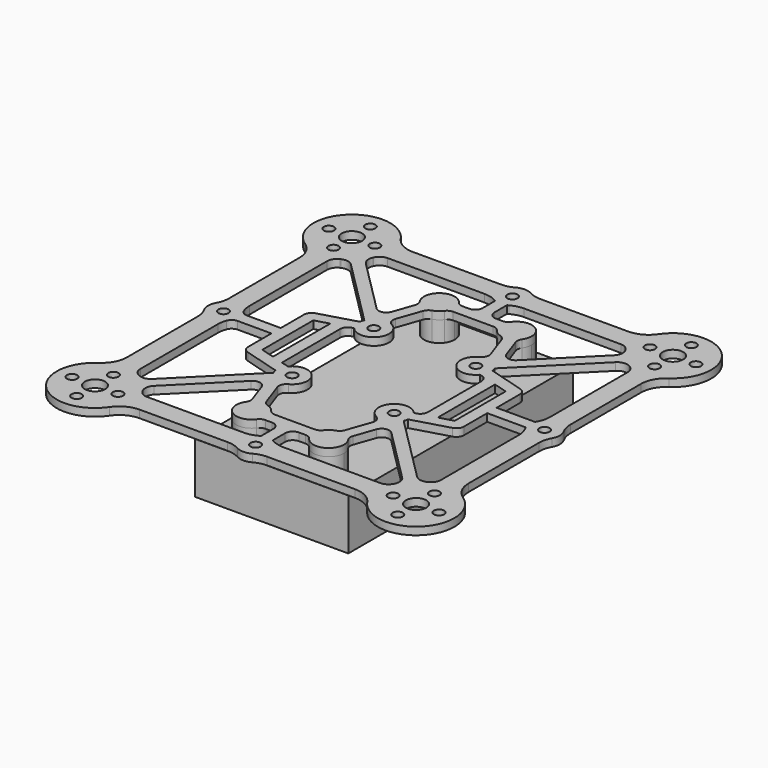
from build123d import *

# Parameters (mm, degrees)
F1_R     = 1
F1_R_2   = 2
F2_DEPTH = 1.5
F4_DEPTH = 4
F5_W     = 30
F5_H     = 55
F5_R     = 3
F6_DEPTH = 10


with BuildPart() as f2:
    # F1 (on Top) → F2 (new body)
    with BuildSketch(Plane.XY):
        with BuildLine():
            ThreePointArc((-33.4662517628, -21.1100941742), (-34.0503713296, -23.4553020541), (-35.6662517628, -25.2525572096))
            ThreePointArc((-35.6662517628, -25.2525572096), (-36.7695526217, -36.7695526217), (-25.2525572096, -35.6662517628))
            ThreePointArc((-25.2525572096, -35.6662517628), (-23.4553020541, -34.0503713296), (-21.1100941742, -33.4662517628))
            Line((-21.1100941742, -33.4662517628), (-3.8729833462, -33.4662517628))
            ThreePointArc((-3.8729833462, -33.4662517628), (-2.6229833462, -33.62502258), (-1.4523687548, -34.0912517628))
            ThreePointArc((-1.4523687548, -34.0912517628), (0, -34.4662517628), (1.4523687548, -34.0912517628))
            ThreePointArc((1.4523687548, -34.0912517628), (2.6229833462, -33.62502258), (3.8729833462, -33.4662517628))
            Line((3.8729833462, -33.4662517628), (21.1100941742, -33.4662517628))
            ThreePointArc((21.1100941742, -33.4662517628), (23.4553020541, -34.0503713296), (25.2525572096, -35.6662517628))
            ThreePointArc((25.2525572096, -35.6662517628), (36.7695526217, -36.7695526217), (35.6662517628, -25.2525572096))
            ThreePointArc((35.6662517628, -25.2525572096), (34.0503713296, -23.4553020541), (33.4662517628, -21.1100941742))
            Line((33.4662517628, -21.1100941742), (33.4662517628, -3.8729833462))
            ThreePointArc((33.4662517628, -3.8729833462), (33.62502258, -2.6229833462), (34.0912517628, -1.4523687548))
            ThreePointArc((34.0912517628, -1.4523687548), (34.4662517628, 0), (34.0912517628, 1.4523687548))
            ThreePointArc((34.0912517628, 1.4523687548), (33.62502258, 2.6229833462), (33.4662517628, 3.8729833462))
            Line((33.4662517628, 3.8729833462), (33.4662517628, 21.1100941742))
            ThreePointArc((33.4662517628, 21.1100941742), (34.0503713296, 23.4553020541), (35.6662517628, 25.2525572096))
            ThreePointArc((35.6662517628, 25.2525572096), (36.7695526217, 36.7695526217), (25.2525572096, 35.6662517628))
            ThreePointArc((25.2525572096, 35.6662517628), (23.4553020541, 34.0503713296), (21.1100941742, 33.4662517628))
            Line((21.1100941742, 33.4662517628), (3.8729833462, 33.4662517628))
            ThreePointArc((3.8729833462, 33.4662517628), (2.6229833462, 33.62502258), (1.4523687548, 34.0912517628))
            ThreePointArc((1.4523687548, 34.0912517628), (0, 34.4662517628), (-1.4523687548, 34.0912517628))
            ThreePointArc((-1.4523687548, 34.0912517628), (-2.6229833462, 33.62502258), (-3.8729833462, 33.4662517628))
            Line((-3.8729833462, 33.4662517628), (-21.1100941742, 33.4662517628))
            ThreePointArc((-21.1100941742, 33.4662517628), (-23.4553020541, 34.0503713296), (-25.2525572096, 35.6662517628))
            ThreePointArc((-25.2525572096, 35.6662517628), (-36.7695526217, 36.7695526217), (-35.6662517628, 25.2525572096))
            ThreePointArc((-35.6662517628, 25.2525572096), (-34.0503713296, 23.4553020541), (-33.4662517628, 21.1100941742))
            Line((-33.4662517628, 21.1100941742), (-33.4662517628, 3.8729833462))
            ThreePointArc((-33.4662517628, 3.8729833462), (-33.62502258, 2.6229833462), (-34.0912517628, 1.4523687548))
            ThreePointArc((-34.0912517628, 1.4523687548), (-34.4662517628, 0), (-34.0912517628, -1.4523687548))
            ThreePointArc((-34.0912517628, -1.4523687548), (-33.62502258, -2.6229833462), (-33.4662517628, -3.8729833462))
            Line((-33.4662517628, -3.8729833462), (-33.4662517628, -21.1100941742))
        make_face()
        with Locations((-31.4662517628, -35.9662517628)):
            Circle(F1_R, mode=Mode.SUBTRACT)
        with Locations((-35.9662517628, -31.4662517628)):
            Circle(F1_R, mode=Mode.SUBTRACT)
        with Locations((-31.4662517628, -31.4662517628)):
            Circle(F1_R_2, mode=Mode.SUBTRACT)
        with Locations((-26.9662517628, -31.4662517628)):
            Circle(F1_R, mode=Mode.SUBTRACT)
        with Locations((-31.4662517628, -26.9662517628)):
            Circle(F1_R, mode=Mode.SUBTRACT)
        with BuildLine():
            ThreePointArc((-22.849407793, -29.4662517628), (-23.9254629667, -29.1521062236), (-24.6634802077, -28.308357026))
            ThreePointArc((-24.6634802077, -28.308357026), (-24.6838554075, -28.2648302537), (-24.7045091049, -28.2214349377))
            ThreePointArc((-24.7045091049, -28.2214349377), (-24.8728885591, -27.0197800467), (-24.3155912919, -25.9419368886))
            Line((-24.3155912919, -25.9419368886), (-13.7338277743, -15.360173371))
            ThreePointArc((-13.7338277743, -15.360173371), (-12.3402923362, -14.9582351505), (-11.257957598, -15.9236608934))
            Line((-11.257957598, -15.9236608934), (-9.8435524525, -19.9497880645))
            ThreePointArc((-9.8435524525, -19.9497880645), (-9.7719536477, -20.6454539498), (-10.0235391122, -21.2979738092))
            ThreePointArc((-10.0235391122, -21.2979738092), (-9.2875900594, -25.4477577388), (-5.1284504101, -24.7666666667))
            ThreePointArc((-5.1284504101, -24.7666666667), (-4.5962029293, -24.3130258043), (-3.9161294039, -24.15))
            Line((-3.9161294039, -24.15), (-2.65, -24.15))
            ThreePointArc((-2.65, -24.15), (-1.5893398282, -24.5893398282), (-1.15, -25.65))
            Line((-1.15, -25.65), (-1.15, -28.6954215623))
            ThreePointArc((-1.15, -28.6954215623), (-1.3032257655, -28.7641039867), (-1.4523687548, -28.8412517628))
            ThreePointArc((-1.4523687548, -28.8412517628), (-2.6229833462, -29.3074809456), (-3.8729833462, -29.4662517628))
            Line((-3.8729833462, -29.4662517628), (-22.849407793, -29.4662517628))
        make_face(mode=Mode.SUBTRACT)
        with BuildLine():
            ThreePointArc((-28.308357026, -24.6634802077), (-29.1521062236, -23.9254629667), (-29.4662517628, -22.849407793))
            Line((-29.4662517628, -22.849407793), (-29.4662517628, -3.8729833462))
            ThreePointArc((-29.4662517628, -3.8729833462), (-29.3868269069, -2.9853233599), (-29.1510756623, -2.1258642802))
            ThreePointArc((-29.1510756623, -2.1258642802), (-28.6011389892, -1.4178872658), (-27.7456284924, -1.15))
            Line((-27.7456284924, -1.15), (-21.15, -1.15))
            Line((-21.15, -1.15), (-21.15, -6.8384922452))
            ThreePointArc((-21.15, -6.8384922452), (-20.8492479119, -7.7394941575), (-20.0675940722, -8.2791917944))
            Line((-20.0675940722, -8.2791917944), (-12.9814446691, -10.3331481431))
            ThreePointArc((-12.9814446691, -10.3331481431), (-12.9055182091, -10.7469698366), (-12.7724456227, -11.1461000259))
            Line((-12.7724456227, -11.1461000259), (-25.9419368886, -24.3155912919))
            ThreePointArc((-25.9419368886, -24.3155912919), (-27.0197800467, -24.8728885591), (-28.2214349377, -24.7045091049))
            ThreePointArc((-28.2214349377, -24.7045091049), (-28.2648302537, -24.6838554075), (-28.308357026, -24.6634802077))
        make_face(mode=Mode.SUBTRACT)
        with Locations((-10, -10)):
            Circle(F1_R, mode=Mode.SUBTRACT)
        Polygon((-18.85, 6.237447605), (-16.15, 7.0200563006), (-16.15, -7.0200563006), (-18.85, -6.237447605), align=None, mode=Mode.SUBTRACT)
        with Locations((0, -31.4662517628)):
            Circle(F1_R, mode=Mode.SUBTRACT)
        with BuildLine():
            ThreePointArc((24.6634802077, -28.308357026), (23.9254629667, -29.1521062236), (22.849407793, -29.4662517628))
            Line((22.849407793, -29.4662517628), (3.8729833462, -29.4662517628))
            ThreePointArc((3.8729833462, -29.4662517628), (2.6229833462, -29.3074809456), (1.4523687548, -28.8412517628))
            ThreePointArc((1.4523687548, -28.8412517628), (1.3032257655, -28.7641039867), (1.15, -28.6954215623))
            Line((1.15, -28.6954215623), (1.15, -25.65))
            ThreePointArc((1.15, -25.65), (1.5893398282, -24.5893398282), (2.65, -24.15))
            Line((2.65, -24.15), (3.9161294039, -24.15))
            ThreePointArc((3.9161294039, -24.15), (4.5962029293, -24.3130258043), (5.1284504101, -24.7666666667))
            ThreePointArc((5.1284504101, -24.7666666667), (9.2875900594, -25.4477577388), (10.0235391122, -21.2979738092))
            ThreePointArc((10.0235391122, -21.2979738092), (9.7719536477, -20.6454539498), (9.8435524525, -19.9497880645))
            Line((9.8435524525, -19.9497880645), (11.257957598, -15.9236608934))
            ThreePointArc((11.257957598, -15.9236608934), (12.3402923362, -14.9582351505), (13.7338277743, -15.360173371))
            Line((13.7338277743, -15.360173371), (24.3155912919, -25.9419368886))
            ThreePointArc((24.3155912919, -25.9419368886), (24.8728885591, -27.0197800467), (24.7045091049, -28.2214349377))
            ThreePointArc((24.7045091049, -28.2214349377), (24.6838554075, -28.2648302537), (24.6634802077, -28.308357026))
        make_face(mode=Mode.SUBTRACT)
        with Locations((26.9662517628, -31.4662517628)):
            Circle(F1_R, mode=Mode.SUBTRACT)
        with Locations((31.4662517628, -35.9662517628)):
            Circle(F1_R, mode=Mode.SUBTRACT)
        with Locations((31.4662517628, -31.4662517628)):
            Circle(F1_R_2, mode=Mode.SUBTRACT)
        with Locations((35.9662517628, -31.4662517628)):
            Circle(F1_R, mode=Mode.SUBTRACT)
        with Locations((31.4662517628, -26.9662517628)):
            Circle(F1_R, mode=Mode.SUBTRACT)
        with Locations((10, -10)):
            Circle(F1_R, mode=Mode.SUBTRACT)
        Polygon((16.15, -7.0200563006), (16.15, 7.0200563006), (18.85, 6.237447605), (18.85, -6.237447605), align=None, mode=Mode.SUBTRACT)
        with BuildLine():
            ThreePointArc((29.4662517628, -22.849407793), (29.1521062236, -23.9254629667), (28.308357026, -24.6634802077))
            ThreePointArc((28.308357026, -24.6634802077), (28.2648302537, -24.6838554075), (28.2214349377, -24.7045091049))
            ThreePointArc((28.2214349377, -24.7045091049), (27.0197800467, -24.8728885591), (25.9419368886, -24.3155912919))
            Line((25.9419368886, -24.3155912919), (12.7724456227, -11.1461000259))
            ThreePointArc((12.7724456227, -11.1461000259), (12.9055182091, -10.7469698366), (12.9814446691, -10.3331481431))
            Line((12.9814446691, -10.3331481431), (20.0675940722, -8.2791917944))
            ThreePointArc((20.0675940722, -8.2791917944), (20.8492479119, -7.7394941575), (21.15, -6.8384922452))
            Line((21.15, -6.8384922452), (21.15, -1.15))
            Line((21.15, -1.15), (28.6954215623, -1.15))
            ThreePointArc((28.6954215623, -1.15), (28.7641039867, -1.3032257655), (28.8412517628, -1.4523687548))
            ThreePointArc((28.8412517628, -1.4523687548), (29.3074809456, -2.6229833462), (29.4662517628, -3.8729833462))
            Line((29.4662517628, -3.8729833462), (29.4662517628, -22.849407793))
        make_face(mode=Mode.SUBTRACT)
        with Locations((-31.4662517628, 0)):
            Circle(F1_R, mode=Mode.SUBTRACT)
        with BuildLine():
            ThreePointArc((-29.4662517628, 22.849407793), (-29.1521062236, 23.9254629667), (-28.308357026, 24.6634802077))
            ThreePointArc((-28.308357026, 24.6634802077), (-28.2648302537, 24.6838554075), (-28.2214349377, 24.7045091049))
            ThreePointArc((-28.2214349377, 24.7045091049), (-27.0197800467, 24.8728885591), (-25.9419368886, 24.3155912919))
            Line((-25.9419368886, 24.3155912919), (-12.7724456227, 11.1461000259))
            ThreePointArc((-12.7724456227, 11.1461000259), (-12.9055182091, 10.7469698366), (-12.9814446691, 10.3331481431))
            Line((-12.9814446691, 10.3331481431), (-20.0675940722, 8.2791917944))
            ThreePointArc((-20.0675940722, 8.2791917944), (-20.8492479119, 7.7394941575), (-21.15, 6.8384922452))
            Line((-21.15, 6.8384922452), (-21.15, 1.15))
            Line((-21.15, 1.15), (-27.7456284924, 1.15))
            ThreePointArc((-27.7456284924, 1.15), (-28.6011389892, 1.4178872658), (-29.1510756623, 2.1258642802))
            ThreePointArc((-29.1510756623, 2.1258642802), (-29.3868269069, 2.9853233599), (-29.4662517628, 3.8729833462))
            Line((-29.4662517628, 3.8729833462), (-29.4662517628, 22.849407793))
        make_face(mode=Mode.SUBTRACT)
        with Locations((-10, 10)):
            Circle(F1_R, mode=Mode.SUBTRACT)
        with Locations((-31.4662517628, 26.9662517628)):
            Circle(F1_R, mode=Mode.SUBTRACT)
        with Locations((-35.9662517628, 31.4662517628)):
            Circle(F1_R, mode=Mode.SUBTRACT)
        with Locations((-31.4662517628, 31.4662517628)):
            Circle(F1_R_2, mode=Mode.SUBTRACT)
        with Locations((-31.4662517628, 35.9662517628)):
            Circle(F1_R, mode=Mode.SUBTRACT)
        with Locations((-26.9662517628, 31.4662517628)):
            Circle(F1_R, mode=Mode.SUBTRACT)
        with BuildLine():
            ThreePointArc((-3.8729833462, 29.4662517628), (-2.6229833462, 29.3074809456), (-1.4523687548, 28.8412517628))
            ThreePointArc((-1.4523687548, 28.8412517628), (-1.3032257655, 28.7641039867), (-1.15, 28.6954215623))
            Line((-1.15, 28.6954215623), (-1.15, 25.65))
            ThreePointArc((-1.15, 25.65), (-1.5893398282, 24.5893398282), (-2.65, 24.15))
            Line((-2.65, 24.15), (-3.9161294039, 24.15))
            ThreePointArc((-3.9161294039, 24.15), (-4.5962029293, 24.3130258043), (-5.1284504101, 24.7666666667))
            ThreePointArc((-5.1284504101, 24.7666666667), (-9.2875900594, 25.4477577388), (-10.0235391122, 21.2979738092))
            ThreePointArc((-10.0235391122, 21.2979738092), (-9.7719536477, 20.6454539498), (-9.8435524525, 19.9497880645))
            Line((-9.8435524525, 19.9497880645), (-11.257957598, 15.9236608934))
            ThreePointArc((-11.257957598, 15.9236608934), (-12.3402923362, 14.9582351505), (-13.7338277743, 15.360173371))
            Line((-13.7338277743, 15.360173371), (-24.3155912919, 25.9419368886))
            ThreePointArc((-24.3155912919, 25.9419368886), (-24.8728885591, 27.0197800467), (-24.7045091049, 28.2214349377))
            ThreePointArc((-24.7045091049, 28.2214349377), (-24.6838554075, 28.2648302537), (-24.6634802077, 28.308357026))
            ThreePointArc((-24.6634802077, 28.308357026), (-23.9254629667, 29.1521062236), (-22.849407793, 29.4662517628))
            Line((-22.849407793, 29.4662517628), (-3.8729833462, 29.4662517628))
        make_face(mode=Mode.SUBTRACT)
        with BuildLine():
            ThreePointArc((9.3262887188, 14.4829483408), (9.3067793127, 13.4362123742), (8.6073858095, 12.6571837943))
            ThreePointArc((8.6073858095, 12.6571837943), (7.6843596907, 8.0926956305), (12.3411337583, 8.1240755011))
            Line((12.3411337583, 8.1240755011), (12.7675940722, 8.0004638159))
            ThreePointArc((12.7675940722, 8.0004638159), (13.5492479119, 7.460766179), (13.85, 6.5597642668))
            Line((13.85, 6.5597642668), (13.85, -6.5597642668))
            ThreePointArc((13.85, -6.5597642668), (13.5492479119, -7.460766179), (12.7675940722, -8.0004638159))
            Line((12.7675940722, -8.0004638159), (12.3411337583, -8.1240755011))
            ThreePointArc((12.3411337583, -8.1240755011), (7.6843596907, -8.0926956305), (8.6073858095, -12.6571837943))
            ThreePointArc((8.6073858095, -12.6571837943), (9.3067793127, -13.4362123742), (9.3262887188, -14.4829483408))
            Line((9.3262887188, -14.4829483408), (7.673563779, -19.1874566688))
            ThreePointArc((7.673563779, -19.1874566688), (7.2943439753, -19.7750532594), (6.6899333239, -20.126856013))
            ThreePointArc((6.6899333239, -20.126856013), (5.8185947859, -20.5522422612), (5.1284504101, -21.2333333333))
            ThreePointArc((5.1284504101, -21.2333333333), (4.5962029293, -21.6869741957), (3.9161294039, -21.85))
            Line((3.9161294039, -21.85), (-3.9161294039, -21.85))
            ThreePointArc((-3.9161294039, -21.85), (-4.5962029293, -21.6869741957), (-5.1284504101, -21.2333333333))
            ThreePointArc((-5.1284504101, -21.2333333333), (-5.8185947859, -20.5522422612), (-6.6899333239, -20.126856013))
            ThreePointArc((-6.6899333239, -20.126856013), (-7.2943439753, -19.7750532594), (-7.673563779, -19.1874566688))
            Line((-7.673563779, -19.1874566688), (-9.3262887188, -14.4829483408))
            ThreePointArc((-9.3262887188, -14.4829483408), (-9.3067793127, -13.4362123742), (-8.6073858095, -12.6571837943))
            ThreePointArc((-8.6073858095, -12.6571837943), (-7.6843596907, -8.0926956305), (-12.3411337583, -8.1240755011))
            Line((-12.3411337583, -8.1240755011), (-13.85, -7.6867229673))
            Line((-13.85, -7.6867229673), (-13.85, 6.5597642668))
            ThreePointArc((-13.85, 6.5597642668), (-13.5492479119, 7.460766179), (-12.7675940722, 8.0004638159))
            Line((-12.7675940722, 8.0004638159), (-12.3411337583, 8.1240755011))
            ThreePointArc((-12.3411337583, 8.1240755011), (-7.6843596907, 8.0926956305), (-8.6073858095, 12.6571837943))
            ThreePointArc((-8.6073858095, 12.6571837943), (-9.3067793127, 13.4362123742), (-9.3262887188, 14.4829483408))
            Line((-9.3262887188, 14.4829483408), (-7.673563779, 19.1874566688))
            ThreePointArc((-7.673563779, 19.1874566688), (-7.2943439753, 19.7750532594), (-6.6899333239, 20.126856013))
            ThreePointArc((-6.6899333239, 20.126856013), (-5.8185947859, 20.5522422612), (-5.1284504101, 21.2333333333))
            ThreePointArc((-5.1284504101, 21.2333333333), (-4.5962029293, 21.6869741957), (-3.9161294039, 21.85))
            Line((-3.9161294039, 21.85), (3.9161294039, 21.85))
            ThreePointArc((3.9161294039, 21.85), (4.5962029293, 21.6869741957), (5.1284504101, 21.2333333333))
            ThreePointArc((5.1284504101, 21.2333333333), (5.8185947859, 20.5522422612), (6.6899333239, 20.126856013))
            ThreePointArc((6.6899333239, 20.126856013), (7.2943439753, 19.7750532594), (7.673563779, 19.1874566688))
            Line((7.673563779, 19.1874566688), (9.3262887188, 14.4829483408))
        make_face(mode=Mode.SUBTRACT)
        with Locations((10, 10)):
            Circle(F1_R, mode=Mode.SUBTRACT)
        with Locations((31.4662517628, 0)):
            Circle(F1_R, mode=Mode.SUBTRACT)
        with BuildLine():
            ThreePointArc((29.4662517628, 3.8729833462), (29.3074809456, 2.6229833462), (28.8412517628, 1.4523687548))
            ThreePointArc((28.8412517628, 1.4523687548), (28.7641039867, 1.3032257655), (28.6954215623, 1.15))
            Line((28.6954215623, 1.15), (21.15, 1.15))
            Line((21.15, 1.15), (21.15, 6.8384922452))
            ThreePointArc((21.15, 6.8384922452), (20.8492479119, 7.7394941575), (20.0675940722, 8.2791917944))
            Line((20.0675940722, 8.2791917944), (12.9814446691, 10.3331481431))
            ThreePointArc((12.9814446691, 10.3331481431), (12.9055182091, 10.7469698366), (12.7724456227, 11.1461000259))
            Line((12.7724456227, 11.1461000259), (25.9419368886, 24.3155912919))
            ThreePointArc((25.9419368886, 24.3155912919), (27.0197800467, 24.8728885591), (28.2214349377, 24.7045091049))
            ThreePointArc((28.2214349377, 24.7045091049), (28.2648302537, 24.6838554075), (28.308357026, 24.6634802077))
            ThreePointArc((28.308357026, 24.6634802077), (29.1521062236, 23.9254629667), (29.4662517628, 22.849407793))
            Line((29.4662517628, 22.849407793), (29.4662517628, 3.8729833462))
        make_face(mode=Mode.SUBTRACT)
        with BuildLine():
            ThreePointArc((22.849407793, 29.4662517628), (23.9254629667, 29.1521062236), (24.6634802077, 28.308357026))
            ThreePointArc((24.6634802077, 28.308357026), (24.6838554075, 28.2648302537), (24.7045091049, 28.2214349377))
            ThreePointArc((24.7045091049, 28.2214349377), (24.8728885591, 27.0197800467), (24.3155912919, 25.9419368886))
            Line((24.3155912919, 25.9419368886), (13.7338277743, 15.360173371))
            ThreePointArc((13.7338277743, 15.360173371), (12.3402923362, 14.9582351505), (11.257957598, 15.9236608934))
            Line((11.257957598, 15.9236608934), (9.8435524525, 19.9497880645))
            ThreePointArc((9.8435524525, 19.9497880645), (9.7719536477, 20.6454539498), (10.0235391122, 21.2979738092))
            ThreePointArc((10.0235391122, 21.2979738092), (9.2875900594, 25.4477577388), (5.1284504101, 24.7666666667))
            ThreePointArc((5.1284504101, 24.7666666667), (4.5962029293, 24.3130258043), (3.9161294039, 24.15))
            Line((3.9161294039, 24.15), (2.65, 24.15))
            ThreePointArc((2.65, 24.15), (1.5893398282, 24.5893398282), (1.15, 25.65))
            Line((1.15, 25.65), (1.15, 28.6954215623))
            ThreePointArc((1.15, 28.6954215623), (1.3032257655, 28.7641039867), (1.4523687548, 28.8412517628))
            ThreePointArc((1.4523687548, 28.8412517628), (2.6229833462, 29.3074809456), (3.8729833462, 29.4662517628))
            Line((3.8729833462, 29.4662517628), (22.849407793, 29.4662517628))
        make_face(mode=Mode.SUBTRACT)
        with Locations((0, 31.4662517628)):
            Circle(F1_R, mode=Mode.SUBTRACT)
        with Locations((31.4662517628, 26.9662517628)):
            Circle(F1_R, mode=Mode.SUBTRACT)
        with Locations((26.9662517628, 31.4662517628)):
            Circle(F1_R, mode=Mode.SUBTRACT)
        with Locations((31.4662517628, 31.4662517628)):
            Circle(F1_R_2, mode=Mode.SUBTRACT)
        with Locations((35.9662517628, 31.4662517628)):
            Circle(F1_R, mode=Mode.SUBTRACT)
        with Locations((31.4662517628, 35.9662517628)):
            Circle(F1_R, mode=Mode.SUBTRACT)
    extrude(amount=F2_DEPTH)


with BuildPart() as f4:
    # F3 (on face) → F4 (new body)
    with BuildSketch(Plane(origin=(0, 0, 0), x_dir=(1, 0, 0), z_dir=(0, 0, -1))):
        with BuildLine():
            ThreePointArc((-5.1284504101, 21.2333333333), (-4.7005561795, 22.071002163), (-4.5530924227, 23))
            ThreePointArc((-4.5530924227, 23), (-4.7005561795, 23.928997837), (-5.1284504101, 24.7666666667))
            ThreePointArc((-5.1284504101, 24.7666666667), (-9.2875900594, 25.4477577388), (-10.0235391122, 21.2979738092))
            ThreePointArc((-10.0235391122, 21.2979738092), (-8.5474377214, 20.1695799911), (-6.6899333239, 20.126856013))
            ThreePointArc((-6.6899333239, 20.126856013), (-5.8185947859, 20.5522422612), (-5.1284504101, 21.2333333333))
        make_face()
    extrude(amount=F4_DEPTH)


with BuildPart() as f4b:
    # F3 (on face) → F4, piece 2 (new body)
    with BuildSketch(Plane(origin=(0, 0, 0), x_dir=(1, 0, 0), z_dir=(0, 0, -1))):
        with BuildLine():
            ThreePointArc((5.1284504101, 24.7666666667), (4.5530924227, 23), (5.1284504101, 21.2333333333))
            ThreePointArc((5.1284504101, 21.2333333333), (5.8185947859, 20.5522422612), (6.6899333239, 20.126856013))
            ThreePointArc((6.6899333239, 20.126856013), (8.5474377214, 20.1695799911), (10.0235391122, 21.2979738092))
            ThreePointArc((10.0235391122, 21.2979738092), (10.4176464952, 22.1087480908), (10.5530924227, 23))
            ThreePointArc((10.5530924227, 23), (8.4820902597, 25.8525362432), (5.1284504101, 24.7666666667))
        make_face()
    extrude(amount=F4_DEPTH)


with BuildPart() as f4c:
    # F3 (on face) → F4, piece 3 (new body)
    with BuildSketch(Plane(origin=(0, 0, 0), x_dir=(1, 0, 0), z_dir=(0, 0, -1))):
        with BuildLine():
            ThreePointArc((-5.1284504101, -21.2333333333), (-5.8185947859, -20.5522422612), (-6.6899333239, -20.126856013))
            ThreePointArc((-6.6899333239, -20.126856013), (-8.5474377214, -20.1695799911), (-10.0235391122, -21.2979738092))
            ThreePointArc((-10.0235391122, -21.2979738092), (-9.2875900594, -25.4477577388), (-5.1284504101, -24.7666666667))
            ThreePointArc((-5.1284504101, -24.7666666667), (-4.7005561795, -23.928997837), (-4.5530924227, -23))
            ThreePointArc((-4.5530924227, -23), (-4.7005561795, -22.071002163), (-5.1284504101, -21.2333333333))
        make_face()
    extrude(amount=F4_DEPTH)


with BuildPart() as f4d:
    # F3 (on face) → F4, piece 4 (new body)
    with BuildSketch(Plane(origin=(0, 0, 0), x_dir=(1, 0, 0), z_dir=(0, 0, -1))):
        with BuildLine():
            ThreePointArc((6.6899333239, -20.126856013), (5.8185947859, -20.5522422612), (5.1284504101, -21.2333333333))
            ThreePointArc((5.1284504101, -21.2333333333), (4.5530924227, -23), (5.1284504101, -24.7666666667))
            ThreePointArc((5.1284504101, -24.7666666667), (8.4820902597, -25.8525362432), (10.5530924227, -23))
            ThreePointArc((10.5530924227, -23), (10.4176464952, -22.1087480908), (10.0235391122, -21.2979738092))
            ThreePointArc((10.0235391122, -21.2979738092), (8.5474377214, -20.1695799911), (6.6899333239, -20.126856013))
        make_face()
    extrude(amount=F4_DEPTH)


with BuildPart() as f6:
    # F5 (on face) → F6 (new body)
    with BuildSketch(Plane(origin=(0, 0, -4), x_dir=(1, 0, 0), z_dir=(0, 0, -1))):
        Rectangle(F5_W, F5_H)
        with Locations((-7.5530924227, 23)):
            Circle(F5_R, mode=Mode.SUBTRACT)
        with Locations((-7.5530924227, 23)):
            Circle(F5_R)
    extrude(amount=F6_DEPTH)


solid = Compound([f2.part, f4.part, f4b.part, f4c.part, f4d.part, f6.part])
